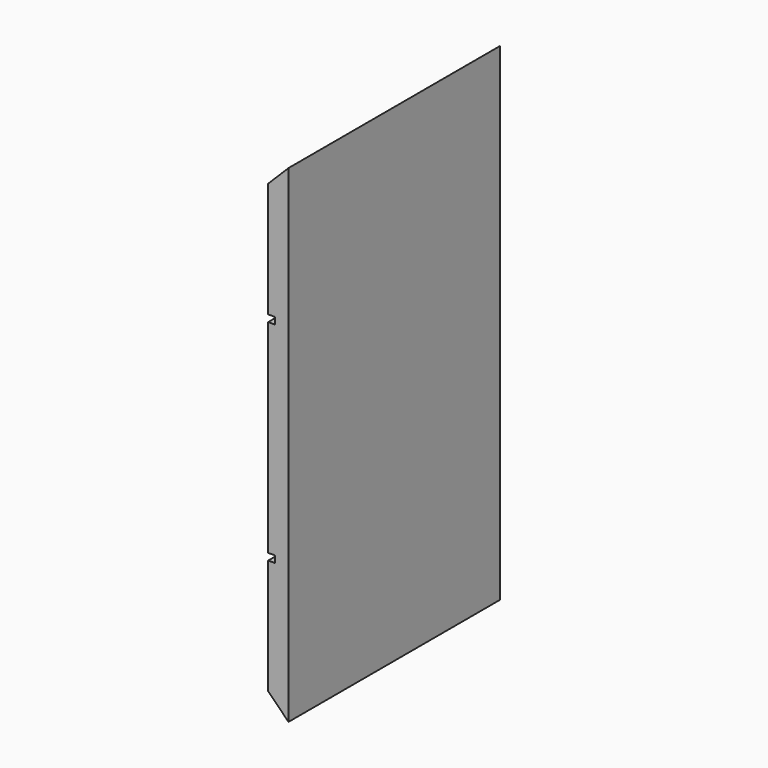
from build123d import *

# Parameters (mm, degrees)
F0_W     = 247.65
F0_H     = 457.2
F1_DEPTH = 19.05
F2_W     = 12.7
F2_H     = 19.05
F3_DEPTH = 457.201
F4_SIZE  = 19.04999
F5_SIZE  = 19.04999
F6_W     = 228.6
F6_H     = 6.35
F7_DEPTH = 6.35


# Not quite as in the source:
# - a fillet or chamfer is up to 0.001 mm smaller than in the source, because OpenCascade refuses the exact size


with BuildPart() as f1:
    # F0 (on Right) → F1 (new body)
    with BuildSketch(Plane.YZ):
        Rectangle(F0_W, F0_H)
    extrude(amount=F1_DEPTH)

    # F2 (on face) → F3 (cut, through all)
    with BuildSketch(Plane(origin=(0, 0, -228.6), x_dir=(1, 0, 0), z_dir=(0, 0, -1))):
        with Locations((6.35, -114.3)):
            Rectangle(F2_W, F2_H)
    extrude(amount=-F3_DEPTH, mode=Mode.SUBTRACT)

    # F4 (size 19.05 in the source; OpenCascade refuses exactly that, so slightly less here)
    f4_edges = [f1.edges().sort_by_distance(p)[0] for p in [
        (0, -9.525, 228.6),
    ]]
    chamfer(f4_edges, length=F4_SIZE)

    # F5 (size 19.05 in the source; OpenCascade refuses exactly that, so slightly less here)
    f5_edges = [f1.edges().sort_by_distance(p)[0] for p in [
        (0, -9.525, -228.6),
    ]]
    chamfer(f5_edges, length=F5_SIZE)

    # F6 (on face) → F7 (cut)
    with BuildSketch(Plane(origin=(0, 0, 0), x_dir=(0, -1, 0), z_dir=(-1, 0, 0))):
        with Locations((9.525, -98.425)):
            Rectangle(F6_W, F6_H)
        with Locations((9.525, 98.425)):
            Rectangle(F6_W, F6_H)
    extrude(amount=-F7_DEPTH, mode=Mode.SUBTRACT)


solid = f1.part
